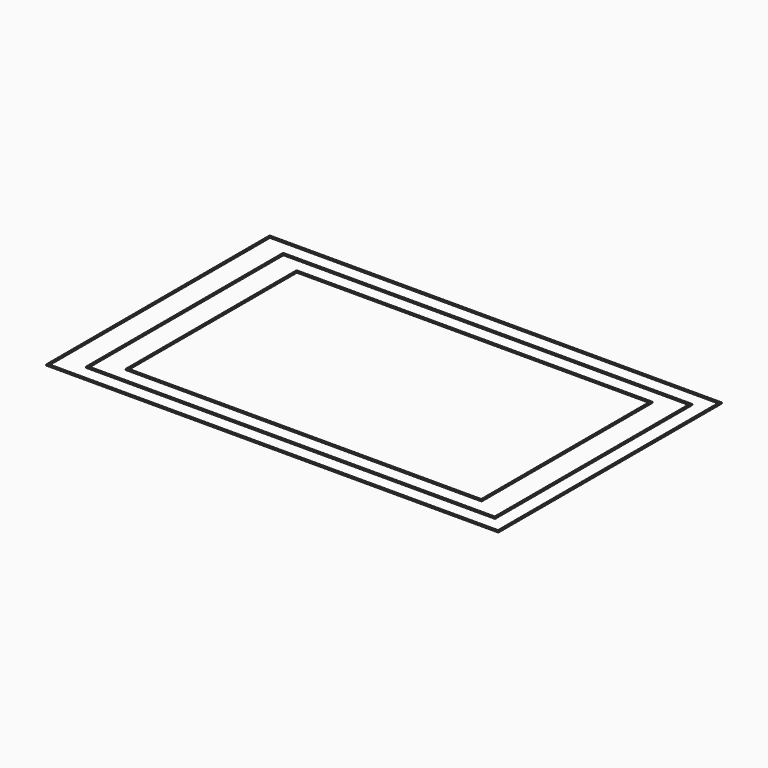
from build123d import *

# Parameters (mm, degrees)
F1_W     = 189.2
F1_H     = 114
F1_W_2   = 187.6
F1_H_2   = 112.4
F2_DEPTH = 0.45
F1_W_3   = 209.1
F1_H_3   = 129.2
F1_W_4   = 207.5
F1_H_4   = 127.6
F1_W_5   = 164.6
F1_H_5   = 98.8
F1_W_6   = 163
F1_H_6   = 97.2


# Not quite as in the source:
# - a feature names something its author has since deleted; it is built from what else it names


with BuildPart() as f2:
    # F1 (on Top) → F2 (new body)
    with BuildSketch(Plane.XY):
        with Locations((15.4175617039, -7.5367691362)):
            Rectangle(F1_W, F1_H)
        with Locations((15.4175617039, -7.5367691362)):
            Rectangle(F1_W_2, F1_H_2, mode=Mode.SUBTRACT)
    extrude(amount=F2_DEPTH)


with BuildPart() as f2b:
    # F1 (on Top) → F2, piece 2 (new body)
    with BuildSketch(Plane.XY):
        with Locations((13.0675617039, -7.5367691362)):
            Rectangle(F1_W_3, F1_H_3)
        with Locations((13.0675617039, -7.5367691362)):
            Rectangle(F1_W_4, F1_H_4, mode=Mode.SUBTRACT)
    extrude(amount=F2_DEPTH)


with BuildPart() as f2c:
    # F1 (on Top) → F2, piece 3 (new body)
    with BuildSketch(Plane.XY):
        with Locations((15.4175617039, -7.5367691362)):
            Rectangle(F1_W_5, F1_H_5)
        with Locations((15.4175617039, -7.5367691362)):
            Rectangle(F1_W_6, F1_H_6, mode=Mode.SUBTRACT)
    extrude(amount=F2_DEPTH)


solid = Compound([f2.part, f2b.part, f2c.part])
